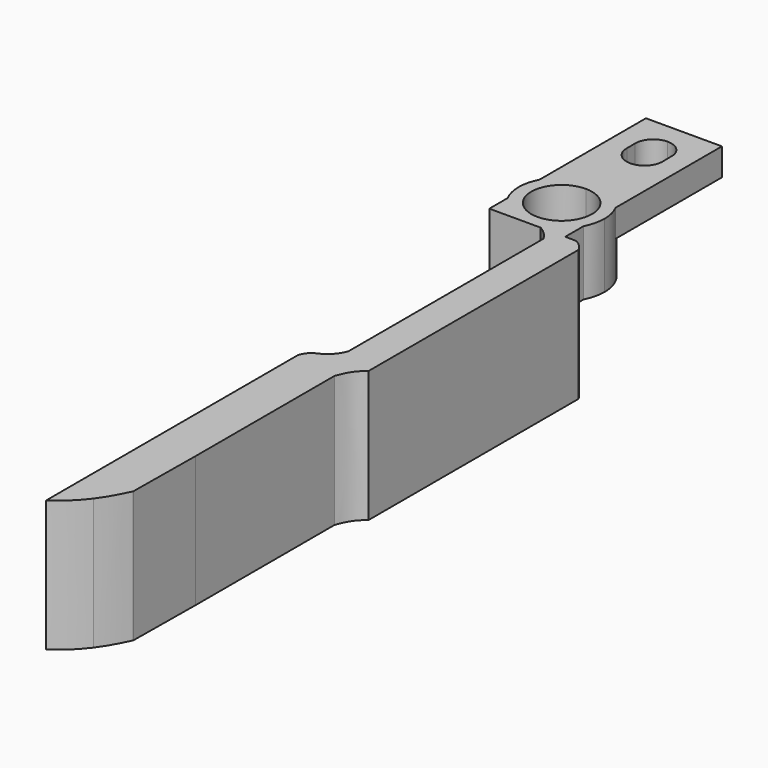
from build123d import *

# Parameters (mm, degrees)
F1_DEPTH = 5.9
F2_DEPTH = 2.5
F3_DEPTH = 12
F4_DEPTH = 12


with BuildPart() as f1:
    # F0 (on Top) → F1 (new body)
    with BuildSketch(Plane.XY):
        with BuildLine():
            Line((0, 2.1001712409), (0, 0))
            Line((0, 0), (1.025, 0))
            Line((1.025, 0), (1.025, 0.8585484677))
            ThreePointArc((1.025, 0.8585484677), (0.4481513041, 1.426237912), (0, 2.1001712409))
        make_face()
        with BuildLine():
            Line((1.025, 0.8585484677), (1.025, 0))
            Line((1.025, 0), (3.475, 0))
            ThreePointArc((3.475, 0), (2.1769624937, 0.2208504846), (1.025, 0.8585484677))
        make_face()
        with BuildLine():
            ThreePointArc((0, 5.7498287591), (-0.45, 3.925), (0, 2.1001712409))
            Line((0, 2.1001712409), (0, 5.7498287591))
        make_face()
        with BuildLine():
            Line((0, 5.7498287591), (0, 2.1001712409))
            ThreePointArc((0, 2.1001712409), (0.4481513041, 1.426237912), (1.025, 0.8585484677))
            ThreePointArc((1.025, 0.8585484677), (2.1769624937, 0.2208504846), (3.475, 0))
            Line((3.475, 0), (3.475, 1.15))
            ThreePointArc((3.475, 1.15), (0.7, 3.925), (3.475, 6.7))
            Line((3.475, 6.7), (3.475, 6.8908035755))
            Line((3.475, 6.8908035755), (3.475, 7.85))
            ThreePointArc((3.475, 7.85), (1.4448310267, 7.2841723593), (0, 5.7498287591))
        make_face()
        with BuildLine():
            ThreePointArc((5.925, 0.8585484677), (4.7730375063, 0.2208504846), (3.475, 0))
            Line((3.475, 0), (4.7, 0))
            Line((4.7, 0), (5.925, 0))
            Line((5.925, 0), (5.925, 0.8585484677))
        make_face()
        with BuildLine():
            Line((3.475, 1.15), (3.475, 0))
            ThreePointArc((3.475, 0), (4.7730375063, 0.2208504846), (5.925, 0.8585484677))
            ThreePointArc((5.925, 0.8585484677), (6.5018486959, 1.426237912), (6.95, 2.1001712409))
            Line((6.95, 2.1001712409), (6.95, 5.7498287591))
            ThreePointArc((6.95, 5.7498287591), (5.5051689733, 7.2841723593), (3.475, 7.85))
            Line((3.475, 7.85), (3.475, 6.8908035755))
            Line((3.475, 6.8908035755), (3.475, 6.7))
            ThreePointArc((3.475, 6.7), (5.4372213178, 5.8872213178), (6.25, 3.925))
            ThreePointArc((6.25, 3.925), (5.4372213178, 1.9627786822), (3.475, 1.15))
        make_face()
        with BuildLine():
            Line((5.925, 0), (4.7, 0))
            add(Edge.make_bspline(
                [(4.7, 0), (5.2537494339, -0.3164176305), (5.6369397789, -0.7196032093), (5.925, -1.225)],
                knots=[0, 0, 0, 0, 1.7324116139, 1.7324116139, 1.7324116139, 1.7324116139], degree=3))
            Line((5.925, -1.225), (5.925, -0.079424061))
            Line((5.925, -0.079424061), (5.925, 0))
        make_face()
        with BuildLine():
            ThreePointArc((6.95, 2.1001712409), (6.5018486959, 1.426237912), (5.925, 0.8585484677))
            Line((5.925, 0.8585484677), (5.925, 0))
            Line((5.925, 0), (6.95, 0))
            Line((6.95, 0), (6.95, 0.75))
            Line((6.95, 0.75), (6.95, 1.44))
            Line((6.95, 1.44), (6.95, 1.5))
            Line((6.95, 1.5), (6.95, 2.1001712409))
        make_face()
        with BuildLine():
            Line((6.95, 5.7498287591), (6.95, 2.1001712409))
            ThreePointArc((6.95, 2.1001712409), (7.2858398025, 2.9852526935), (7.4, 3.925))
            ThreePointArc((7.4, 3.925), (7.2858398025, 4.8647473065), (6.95, 5.7498287591))
        make_face()
    extrude(amount=-F1_DEPTH)

    # F0 (on Top) → F2 (join)
    with BuildSketch(Plane.XY):
        with BuildLine():
            Line((0, 7.85), (0, 5.7498287591))
            ThreePointArc((0, 5.7498287591), (1.4448310267, 7.2841723593), (3.475, 7.85))
            ThreePointArc((3.475, 7.85), (5.5051689733, 7.2841723593), (6.95, 5.7498287591))
            Line((6.95, 5.7498287591), (6.95, 17.9))
            Line((6.95, 17.9), (3.475, 17.9))
            Line((3.475, 17.9), (0, 17.9))
            Line((0, 17.9), (0, 7.85))
        make_face()
        with BuildLine():
            ThreePointArc((1.8276640256, 14.3833613398), (2.3042302705, 15.55900427), (3.475, 16.0474200003))
            ThreePointArc((3.475, 16.0474200003), (4.5253988967, 15.6691157612), (5.0933824344, 14.7079463483))
            Line((5.0933824344, 14.7079463483), (5.1024433757, 14.1442252627))
            Line((5.1024433757, 14.1442252627), (5.113982201, 13.4263440945))
            ThreePointArc((5.113982201, 13.4263440945), (5.1141409801, 13.4131724726), (5.1141939076, 13.4))
            ThreePointArc((5.1141939076, 13.4), (4.6340851277, 12.2409148723), (3.475, 11.7608060924))
            ThreePointArc((3.475, 11.7608060924), (2.2942628451, 12.2629791393), (1.8369719791, 13.4618131819))
            Line((1.8369719791, 13.4618131819), (1.8276640256, 14.3833613398))
        make_face(mode=Mode.SUBTRACT)
    extrude(amount=-F2_DEPTH)

    # F0 (on Top) → F3 (join)
    with BuildSketch(Plane.XY):
        with BuildLine():
            Line((6.95, 0), (5.925, 0))
            Line((5.925, 0), (5.925, -0.079424061))
            Line((5.925, -0.079424061), (5.925, -1.225))
            Line((5.925, -1.225), (5.925, -21.3844068348))
            Line((5.925, -21.3844068348), (5.925, -22.55))
            Line((5.925, -22.55), (5.925, -22.9875))
            Line((5.925, -22.9875), (5.925, -23.5205553472))
            Line((5.925, -23.5205553472), (5.925, -25))
            Line((5.925, -25), (7.525, -25))
            Line((7.525, -25), (8.9492390995, -25))
            Line((8.9492390995, -25), (8.9492390995, -0.9913714603))
            add(Edge.make_bspline(
                [(7.9496195498, -0.0275818011), (8.4295123816, -0.2455351059), (8.7658986449, -0.6068330258), (8.9492390995, -0.9913714603)],
                knots=[0, 0, 0, 0, 1.3885711186, 1.3885711186, 1.3885711186, 1.3885711186], degree=3))
            Line((7.9496195498, -0.0275818011), (6.95, 0))
        make_face()
        with BuildLine():
            add(Edge.make_bspline(
                [(4.7, -25), (4.0586842224, -25.2618398517), (3.6450892221, -25.6055109203), (3.475, -26.225)],
                knots=[0, 0, 0, 0, 1.7324116139, 1.7324116139, 1.7324116139, 1.7324116139], degree=3))
            Line((3.475, -26.225), (3.475, -48.775))
            Line((3.475, -48.775), (3.475, -50))
            Line((3.475, -50), (5.925, -50))
            Line((5.925, -50), (5.925, -47.55))
            Line((5.925, -47.55), (5.925, -43))
            Line((5.925, -43), (5.925, -28.903))
            Line((5.925, -28.903), (5.925, -26.9515))
            Line((5.925, -26.9515), (5.925, -25))
            Line((5.925, -25), (4.7, -25))
        make_face()
        with BuildLine():
            add(Edge.make_bspline(
                [(4.7, -25), (5.3314492106, -24.6048551053), (5.6424522772, -24.1878218949), (5.925, -23.5205553472)],
                knots=[0, 0, 0, 0, 1.9207762703, 1.9207762703, 1.9207762703, 1.9207762703], degree=3))
            Line((4.7, -25), (5.925, -25))
            Line((5.925, -25), (5.925, -23.5205553472))
        make_face()
        Polygon((7.525, -25), (5.925, -25), (5.925, -26.9515), (5.925, -28.903), (5.925, -43), (7.525, -43), (7.525, -27.1006729454), align=None)
        with BuildLine():
            add(Edge.make_bspline(
                [(8.9492390995, -25), (8.2447035238, -25.5232192576), (7.9111177474, -26.03264153), (7.525, -27.1006729454)],
                knots=[0, 0, 0, 0, 2.5379684466, 2.5379684466, 2.5379684466, 2.5379684466], degree=3))
            Line((8.9492390995, -25), (7.525, -25))
            Line((7.525, -25), (7.525, -27.1006729454))
        make_face()
        with BuildLine():
            Line((5.925, -50), (3.475, -50))
            Line((3.475, -50), (3.475, -55))
            add(Edge.make_bspline(
                [(3.475, -55), (4.512583722, -54.3078648135), (5.2908616095, -53.5264365704), (5.925, -52.6706067544)],
                knots=[0, 0, 0, 0, 3.2551675464, 3.2551675464, 3.2551675464, 3.2551675464], degree=3))
            Line((5.925, -52.6706067544), (5.925, -52.0125))
            Line((5.925, -52.0125), (5.925, -50))
        make_face()
        with BuildLine():
            Line((7.4536274492, -50.0155514561), (5.925, -50))
            Line((5.925, -50), (5.925, -52.0125))
            Line((5.925, -52.0125), (5.925, -52.6706067544))
            add(Edge.make_bspline(
                [(5.925, -52.6706067544), (6.5332867434, -51.8496661845), (7.0089465882, -50.9602665865), (7.4536274492, -50.0155514561)],
                knots=[3.2551675464, 3.2551675464, 3.2551675464, 3.2551675464, 6.3776330772, 6.3776330772, 6.3776330772, 6.3776330772], degree=3))
        make_face()
        Polygon((5.925, -47.55), (5.925, -50), (7.4537856616, -50), (7.525, -43), (5.925, -43), align=None)
    extrude(amount=-F3_DEPTH)

    # F0 (on Top) → F4 (join)
    with BuildSketch(Plane.XY):
        Polygon((7.4537856616, -50), (5.925, -50), (7.4536274492, -50.0155514561), align=None)
    extrude(amount=-F4_DEPTH)


solid = f1.part
